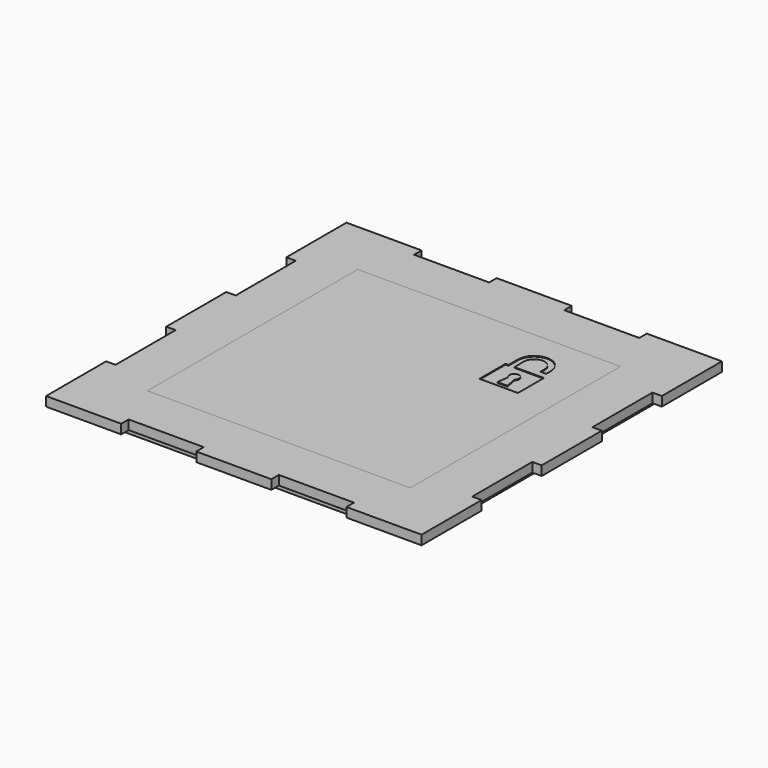
from build123d import *

# Parameters (mm, degrees)
F0_W      = 3.175
F0_H      = 3.175
F0_W_2    = 22.225
F0_W_3    = 25.4
F0_H_2    = 22.225
F0_H_3    = 25.4
F1_DEPTH  = 3.175
F2_W      = 88.9
F2_H      = 88.9
F3_DEPTH  = 25.4
F4_W      = 88.9
F4_H      = 88.9
F5_DEPTH  = 3.175
F6_W      = 114.3
F6_H      = 114.3
F6_W_2    = 76.2
F6_H_2    = 76.2
F7_DEPTH  = 3.175
F8_R      = 36.83
F9_DEPTH  = 3.175
F11_DEPTH = 3.175
F12_R     = 1.5875
F13_DEPTH = 25.4
F14_R     = 8.2290520425
F14_R_2   = 2.2992532289
F15_DEPTH = 1.5875
F16_COUNT = 4
F18_DEPTH = 0.254


with BuildPart() as f1:
    # F0 (on Top) → F1 (new body)
    with BuildSketch(Plane.XY):
        with Locations((-61.9125, 61.9125)):
            Rectangle(F0_W, F0_H)
        with Locations((61.9125, 61.9125)):
            Rectangle(F0_W, F0_H)
        with Locations((-61.9125, -61.9125)):
            Rectangle(F0_W, F0_H)
        with Locations((61.9125, -61.9125)):
            Rectangle(F0_W, F0_H)
        with Locations((-49.2125, 61.9125)):
            Rectangle(F0_W_2, F0_H)
        with Locations((0, 61.9125)):
            Rectangle(F0_W_3, F0_H)
        with Locations((49.2125, 61.9125)):
            Rectangle(F0_W_2, F0_H)
        with Locations((-49.2125, -61.9125)):
            Rectangle(F0_W_2, F0_H)
        with Locations((0, -61.9125)):
            Rectangle(F0_W_3, F0_H)
        with Locations((49.2125, -61.9125)):
            Rectangle(F0_W_2, F0_H)
        with Locations((-61.9125, 49.2125)):
            Rectangle(F0_W, F0_H_2)
        with Locations((-61.9125, 0)):
            Rectangle(F0_W, F0_H_3)
        with Locations((-61.9125, -49.2125)):
            Rectangle(F0_W, F0_H_2)
        with Locations((61.9125, 49.2125)):
            Rectangle(F0_W, F0_H_2)
        with Locations((61.9125, 0)):
            Rectangle(F0_W, F0_H_3)
        with Locations((61.9125, -49.2125)):
            Rectangle(F0_W, F0_H_2)
        with Locations((-49.2125, 49.2125)):
            Rectangle(F0_W_2, F0_H_2)
        with Locations((-25.4, 49.2125)):
            Rectangle(F0_W_3, F0_H_2)
        with Locations((25.4, 49.2125)):
            Rectangle(F0_W_3, F0_H_2)
        with Locations((49.2125, 49.2125)):
            Rectangle(F0_W_2, F0_H_2)
        with Locations((49.2125, 25.4)):
            Rectangle(F0_W_2, F0_H_3)
        with Locations((25.4, 25.4)):
            Rectangle(F0_W_3, F0_H_3)
        with Locations((0, 25.4)):
            Rectangle(F0_W_3, F0_H_3)
        with Locations((-25.4, 25.4)):
            Rectangle(F0_W_3, F0_H_3)
        with Locations((-49.2125, 25.4)):
            Rectangle(F0_W_2, F0_H_3)
        with Locations((-49.2125, 0)):
            Rectangle(F0_W_2, F0_H_3)
        with Locations((-25.4, 0)):
            Rectangle(F0_W_3, F0_H_3)
        Rectangle(F0_W_3, F0_H_3)
        with Locations((25.4, 0)):
            Rectangle(F0_W_3, F0_H_3)
        with Locations((49.2125, 0)):
            Rectangle(F0_W_2, F0_H_3)
        with Locations((49.2125, -25.4)):
            Rectangle(F0_W_2, F0_H_3)
        with Locations((25.4, -25.4)):
            Rectangle(F0_W_3, F0_H_3)
        with Locations((0, -25.4)):
            Rectangle(F0_W_3, F0_H_3)
        with Locations((-25.4, -25.4)):
            Rectangle(F0_W_3, F0_H_3)
        with Locations((-49.2125, -25.4)):
            Rectangle(F0_W_2, F0_H_3)
        with Locations((-49.2125, -49.2125)):
            Rectangle(F0_W_2, F0_H_2)
        with Locations((-25.4, -49.2125)):
            Rectangle(F0_W_3, F0_H_2)
        with Locations((25.4, -49.2125)):
            Rectangle(F0_W_3, F0_H_2)
        with Locations((49.2125, -49.2125)):
            Rectangle(F0_W_2, F0_H_2)
        with Locations((0, 49.2125)):
            Rectangle(F0_W_3, F0_H_2)
        with Locations((0, -49.2125)):
            Rectangle(F0_W_3, F0_H_2)
    extrude(amount=F1_DEPTH)

    # F2 (on face) → F3 (cut)
    with BuildSketch(Plane.XY.offset(3.175)):
        Rectangle(F2_W, F2_H)
    extrude(amount=-F3_DEPTH, mode=Mode.SUBTRACT)


with BuildPart() as f5:
    # F4 (on Top) → F5 (new body)
    with BuildSketch(Plane.XY):
        Rectangle(F4_W, F4_H)
    extrude(amount=F5_DEPTH)

    # F17 (on face) → F18 (cut)
    with BuildSketch(Plane.XY.offset(3.175)):
        Polygon((20.7603132699, 26.7105139792), (19.7496246547, 26.7105139792), (19.7496246547, 15.7025884837), (32.7405332299, 15.7025884837), (32.7405332299, 26.7105139792), (22.7956574124, 26.7105139792), align=None)
        with BuildLine():
            ThreePointArc((25.1143433757, 21.1661748297), (25.5517385216, 23.8284931082), (27.8116554374, 22.3547127098))
            ThreePointArc((27.8116554374, 22.3547127098), (27.6615445924, 21.6757592497), (27.2391947679, 21.123371983))
            Line((27.2391947679, 21.123371983), (27.9931295663, 17.2027479857))
            Line((27.9931295663, 17.2027479857), (24.5691537857, 17.2027479857))
            Line((24.5691537857, 17.2027479857), (25.1143433757, 21.1661748297))
        make_face(mode=Mode.SUBTRACT)
        with BuildLine():
            Line((20.7603132699, 30.6103563624), (20.7603132699, 26.7105139792))
            Line((20.7603132699, 26.7105139792), (22.7956574124, 26.7105139792))
            Line((22.7956574124, 26.7105139792), (22.7223147487, 30.783583757))
            ThreePointArc((22.7223147487, 30.783583757), (26.2883890622, 34.220532707), (29.7689077543, 30.6969700597))
            Line((29.7689077543, 30.6969700597), (29.7689077543, 28.9081595838))
            Line((29.7689077543, 28.9081595838), (31.7305284601, 28.9081595838))
            Line((31.7305284601, 28.9081595838), (31.7305284601, 30.6969700597))
            ThreePointArc((31.7305284601, 30.6969700597), (26.2017707438, 36.1822486135), (20.7603132699, 30.6103563624))
        make_face()
    extrude(amount=-F18_DEPTH, mode=Mode.SUBTRACT)


with BuildPart() as f7:
    # F6 (on face) → F7 (new body)
    with BuildSketch(Plane(origin=(0, 0, 0), x_dir=(1, 0, 0), z_dir=(0, 0, -1))):
        Rectangle(F6_W, F6_H)
        Rectangle(F6_W_2, F6_H_2, mode=Mode.SUBTRACT)
    extrude(amount=F7_DEPTH)


with BuildPart() as f9:
    # F8 (on face) → F9 (new body)
    with BuildSketch(Plane(origin=(0, 0, 0), x_dir=(1, 0, 0), z_dir=(0, 0, -1))):
        Circle(F8_R)
    extrude(amount=F9_DEPTH)


with BuildPart() as f11:
    # F10 (on face) → F11 (new body)
    with BuildSketch(Plane(origin=(0, 0, -3.175), x_dir=(1, 0, 0), z_dir=(0, 0, -1))):
        with BuildLine():
            ThreePointArc((33.6516098645, -14.9672326611), (36.0266407767, -7.6504937322), (36.83, 0))
            ThreePointArc((36.83, 0), (36.0266407721, 7.6504937538), (33.6516098465, 14.9672327015))
            ThreePointArc((33.6516098465, 14.9672327015), (32.7984489867, 16.7544216273), (31.8504573185, 18.4931681602))
            ThreePointArc((31.8504573185, 18.4931681602), (19.3075506603, 19.3075506603), (18.4931681602, 31.8504573185))
            ThreePointArc((18.4931681602, 31.8504573185), (16.7544215813, 32.7984490102), (14.9672326073, 33.6516098884))
            ThreePointArc((14.9672326073, 33.6516098884), (-1e-10, 36.83), (-14.9672326074, 33.6516098883))
            ThreePointArc((-14.9672326074, 33.6516098883), (-16.7544215814, 32.7984490102), (-18.4931681602, 31.8504573185))
            ThreePointArc((-18.4931681602, 31.8504573185), (-17.0251121594, 29.1099831249), (-16.5177427511, 26.0427427511))
            ThreePointArc((-16.5177427511, 26.0427427511), (-17.2427902039, 22.3976830578), (-19.3075506603, 19.3075506603))
            ThreePointArc((-19.3075506603, 19.3075506603), (-25.4256055271, 16.5377563415), (-31.8504573185, 18.4931681602))
            ThreePointArc((-31.8504573185, 18.4931681602), (-32.7984490153, 16.7544215714), (-33.6516098975, 14.9672325869))
            ThreePointArc((-33.6516098975, 14.9672325869), (-36.83, -5.89e-08), (-33.6516098496, -14.9672326945))
            ThreePointArc((-33.6516098496, -14.9672326945), (-32.7984489885, -16.7544216238), (-31.8504573185, -18.4931681602))
            ThreePointArc((-31.8504573185, -18.4931681602), (-21.8351814773, -17.4974485416), (-16.5177427511, -26.0427427511))
            ThreePointArc((-16.5177427511, -26.0427427511), (-17.0251121594, -29.1099831249), (-18.4931681602, -31.8504573185))
            ThreePointArc((-18.4931681602, -31.8504573185), (-16.7544216446, -32.7984489779), (-14.9672327371, -33.6516098306))
            ThreePointArc((-14.9672327371, -33.6516098306), (-9.7e-09, -36.83), (14.9672327195, -33.6516098385))
            ThreePointArc((14.9672327195, -33.6516098385), (16.754421636, -32.7984489823), (18.4931681602, -31.8504573185))
            ThreePointArc((18.4931681602, -31.8504573185), (19.3075506603, -19.3075506603), (31.8504573185, -18.4931681602))
            ThreePointArc((31.8504573185, -18.4931681602), (32.7984489968, -16.7544216075), (33.6516098645, -14.9672326611))
        make_face()
        with BuildLine():
            ThreePointArc((-16.5177427511, 26.0427427511), (-17.0251121594, 29.1099831249), (-18.4931681602, 31.8504573185))
            ThreePointArc((-18.4931681602, 31.8504573185), (-22.4564963273, 29.1916884181), (-26.0427427511, 26.0427427511))
            Line((-26.0427427511, 26.0427427511), (-19.3075506603, 19.3075506603))
            ThreePointArc((-19.3075506603, 19.3075506603), (-17.2427902039, 22.3976830578), (-16.5177427511, 26.0427427511))
        make_face()
        with BuildLine():
            Line((-19.3075506603, 19.3075506603), (-26.0427427511, 26.0427427511))
            ThreePointArc((-26.0427427511, 26.0427427511), (-29.1916884181, 22.4564963273), (-31.8504573185, 18.4931681602))
            ThreePointArc((-31.8504573185, 18.4931681602), (-25.4256055271, 16.5377563415), (-19.3075506603, 19.3075506603))
        make_face()
        with BuildLine():
            ThreePointArc((-31.8504573185, -18.4931681602), (-26.0427427511, -26.0427427511), (-18.4931681602, -31.8504573185))
            ThreePointArc((-18.4931681602, -31.8504573185), (-17.0251121594, -29.1099831249), (-16.5177427511, -26.0427427511))
            ThreePointArc((-16.5177427511, -26.0427427511), (-21.8351814773, -17.4974485416), (-31.8504573185, -18.4931681602))
        make_face()
        with BuildLine():
            ThreePointArc((18.4931681602, -31.8504573185), (26.0427427511, -26.0427427511), (31.8504573185, -18.4931681602))
            ThreePointArc((31.8504573185, -18.4931681602), (19.3075506603, -19.3075506603), (18.4931681602, -31.8504573185))
        make_face()
        with BuildLine():
            ThreePointArc((18.4931681602, 31.8504573185), (19.3075506603, 19.3075506603), (31.8504573185, 18.4931681602))
            ThreePointArc((31.8504573185, 18.4931681602), (26.0427427511, 26.0427427511), (18.4931681602, 31.8504573185))
        make_face()
        with BuildLine():
            ThreePointArc((18.4931681602, 31.8504573185), (26.0427427511, 26.0427427511), (31.8504573185, 18.4931681602))
            ThreePointArc((31.8504573185, 18.4931681602), (33.0775687633, 19.6211504269), (34.0892639218, 20.9457709001))
            ThreePointArc((34.0892639218, 20.9457709001), (35.190658884, 23.3892063514), (35.5677427511, 26.0427427511))
            ThreePointArc((35.5677427511, 26.0427427511), (30.6349628367, 34.3876297896), (20.9457711637, 34.0892640887))
            ThreePointArc((20.9457711637, 34.0892640887), (19.6211505421, 33.0775688685), (18.4931681602, 31.8504573185))
        make_face()
        with BuildLine():
            ThreePointArc((-31.8504573185, 18.4931681602), (-29.1916884181, 22.4564963273), (-26.0427427511, 26.0427427511))
            Line((-26.0427427511, 26.0427427511), (-32.7779348419, 32.7779348419))
            ThreePointArc((-32.7779348419, 32.7779348419), (-35.5097796287, 27.0919509089), (-34.0892641173, 20.9457712087))
            ThreePointArc((-34.0892641173, 20.9457712087), (-33.0775688864, 19.6211505618), (-31.8504573185, 18.4931681602))
        make_face()
        with BuildLine():
            ThreePointArc((-26.0427427511, 26.0427427511), (-22.4564963273, 29.1916884181), (-18.4931681602, 31.8504573185))
            ThreePointArc((-18.4931681602, 31.8504573185), (-19.6211504269, 33.0775687633), (-20.9457709001, 34.0892639218))
            ThreePointArc((-20.9457709001, 34.0892639218), (-27.0919507273, 35.5097796488), (-32.7779348419, 32.7779348419))
            Line((-32.7779348419, 32.7779348419), (-26.0427427511, 26.0427427511))
        make_face()
        with BuildLine():
            ThreePointArc((-20.9457710908, -34.0892640426), (-19.6211505103, -33.0775688394), (-18.4931681602, -31.8504573185))
            ThreePointArc((-18.4931681602, -31.8504573185), (-26.0427427511, -26.0427427511), (-31.8504573185, -18.4931681602))
            ThreePointArc((-31.8504573185, -18.4931681602), (-33.0775688394, -19.6211505103), (-34.0892640426, -20.9457710908))
            ThreePointArc((-34.0892640426, -20.9457710908), (-32.7779348419, -32.7779348419), (-20.9457710908, -34.0892640426))
        make_face()
        with BuildLine():
            ThreePointArc((34.0892640426, -20.9457710908), (33.0775688394, -19.6211505103), (31.8504573185, -18.4931681602))
            ThreePointArc((31.8504573185, -18.4931681602), (26.0427427511, -26.0427427511), (18.4931681602, -31.8504573185))
            ThreePointArc((18.4931681602, -31.8504573185), (19.6211504269, -33.0775687633), (20.9457709001, -34.0892639218))
            ThreePointArc((20.9457709001, -34.0892639218), (30.6349627, -34.3876298648), (35.5677427511, -26.0427427511))
            ThreePointArc((35.5677427511, -26.0427427511), (35.1906589155, -23.3892064598), (34.0892640426, -20.9457710908))
        make_face()
        with BuildLine():
            ThreePointArc((31.8504573185, 18.4931681602), (32.7984489867, 16.7544216273), (33.6516098465, 14.9672327015))
            ThreePointArc((33.6516098465, 14.9672327015), (33.1205578585, 18.0113960911), (34.0892639218, 20.9457709001))
            ThreePointArc((34.0892639218, 20.9457709001), (33.0775687633, 19.6211504269), (31.8504573185, 18.4931681602))
        make_face()
        with BuildLine():
            ThreePointArc((14.9672326073, 33.6516098884), (16.7544215813, 32.7984490102), (18.4931681602, 31.8504573185))
            ThreePointArc((18.4931681602, 31.8504573185), (19.6211505421, 33.0775688685), (20.9457711637, 34.0892640887))
            ThreePointArc((20.9457711637, 34.0892640887), (18.0113961953, 33.1205578662), (14.9672326073, 33.6516098884))
        make_face()
        with BuildLine():
            ThreePointArc((-33.6516098975, 14.9672325869), (-32.7984490153, 16.7544215714), (-31.8504573185, 18.4931681602))
            ThreePointArc((-31.8504573185, 18.4931681602), (-33.0775688864, 19.6211505618), (-34.0892641173, 20.9457712087))
            ThreePointArc((-34.0892641173, 20.9457712087), (-33.3550008175, 19.316814249), (-33.1036115758, 17.5477899927))
            ThreePointArc((-33.1036115758, 17.5477899927), (-33.2421217924, 16.2287393222), (-33.6516098975, 14.9672325869))
        make_face()
        with BuildLine():
            ThreePointArc((-18.4931681602, 31.8504573185), (-16.7544215814, 32.7984490102), (-14.9672326074, 33.6516098883))
            ThreePointArc((-14.9672326074, 33.6516098883), (-18.0113960397, 33.1205578548), (-20.9457709001, 34.0892639218))
            ThreePointArc((-20.9457709001, 34.0892639218), (-19.6211504269, 33.0775687633), (-18.4931681602, 31.8504573185))
        make_face()
        with BuildLine():
            ThreePointArc((-34.0892640426, -20.9457710908), (-33.0775688394, -19.6211505103), (-31.8504573185, -18.4931681602))
            ThreePointArc((-31.8504573185, -18.4931681602), (-32.7984489885, -16.7544216238), (-33.6516098496, -14.9672326945))
            ThreePointArc((-33.6516098496, -14.9672326945), (-33.2421217802, -16.2287393798), (-33.1036115758, -17.5477899927))
            ThreePointArc((-33.1036115758, -17.5477899927), (-33.3550007981, -19.3168141819), (-34.0892640426, -20.9457710908))
        make_face()
        with BuildLine():
            ThreePointArc((-20.9457710908, -34.0892640426), (-18.0113962231, -33.1205578682), (-14.9672327371, -33.6516098306))
            ThreePointArc((-14.9672327371, -33.6516098306), (-16.7544216446, -32.7984489779), (-18.4931681602, -31.8504573185))
            ThreePointArc((-18.4931681602, -31.8504573185), (-19.6211505103, -33.0775688394), (-20.9457710908, -34.0892640426))
        make_face()
        with BuildLine():
            ThreePointArc((20.9457709001, -34.0892639218), (19.6211504269, -33.0775687633), (18.4931681602, -31.8504573185))
            ThreePointArc((18.4931681602, -31.8504573185), (16.754421636, -32.7984489823), (14.9672327195, -33.6516098385))
            ThreePointArc((14.9672327195, -33.6516098385), (18.0113961009, -33.1205578592), (20.9457709001, -34.0892639218))
        make_face()
        with BuildLine():
            ThreePointArc((34.0892640426, -20.9457710908), (33.1205578652, -18.0113961816), (33.6516098645, -14.9672326611))
            ThreePointArc((33.6516098645, -14.9672326611), (32.7984489968, -16.7544216075), (31.8504573185, -18.4931681602))
            ThreePointArc((31.8504573185, -18.4931681602), (33.0775688394, -19.6211505103), (34.0892640426, -20.9457710908))
        make_face()
    extrude(amount=F11_DEPTH)

    # F12 (on face) → F13 (cut)
    with BuildSketch(Plane(origin=(0, 0, -6.35), x_dir=(1, 0, 0), z_dir=(0, 0, -1))):
        Circle(F12_R)
    extrude(amount=-F13_DEPTH, mode=Mode.SUBTRACT)


with BuildPart() as f15:
    # F14 (on face) → F15 (new body)
    with BuildSketch(Plane(origin=(0, 0, -6.35), x_dir=(1, 0, 0), z_dir=(0, 0, -1))):
        with Locations((-26.0427427511, 26.0427427511)):
            Circle(F14_R)
        with Locations((-26.0427427511, 26.0427427511)):
            Circle(F14_R_2, mode=Mode.SUBTRACT)
    extrude(amount=F15_DEPTH)


with BuildPart() as f16_1:
    # F16: instance of F15
    add(f15.part.rotate(Axis((0, 0, -3.175), (0, 0, 1)), 1 * 360 / F16_COUNT))


with BuildPart() as f16_2:
    # F16: instance of F15
    add(f15.part.rotate(Axis((0, 0, -3.175), (0, 0, 1)), 2 * 360 / F16_COUNT))


with BuildPart() as f16_3:
    # F16: instance of F15
    add(f15.part.rotate(Axis((0, 0, -3.175), (0, 0, 1)), 3 * 360 / F16_COUNT))


solid = Compound([f1.part, f5.part, f7.part, f9.part, f11.part, f15.part, f16_1.part, f16_2.part, f16_3.part])
